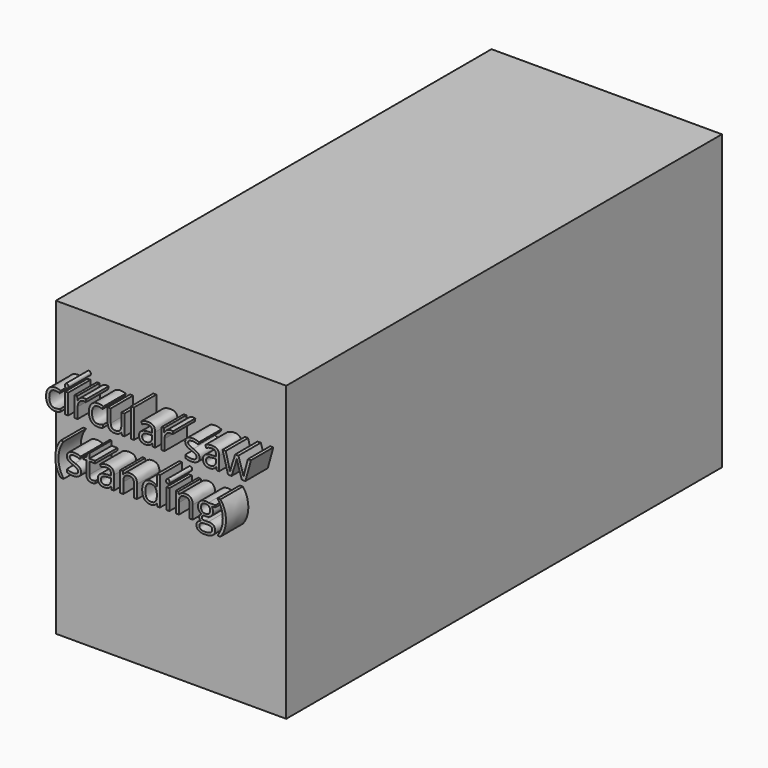
from build123d import *

# Parameters (mm, degrees)
F0_W         = 209.55
F0_H         = 266.7
F1_DEPTH     = 495.3
F2_TEXT_SIZE = 34.2049152733
F3_DEPTH     = 25.4


# Not quite as in the source:
# - Text() gives the source's letters only with a copy of the font that has no kerning and outlines rounded to 1/6400 em; it was checked with that copy


with BuildPart() as f1:
    # F0 (on Front) → F1 (new body)
    with BuildSketch(Plane.XZ):
        Rectangle(F0_W, F0_H)
    extrude(amount=F1_DEPTH)

    # F2 (on face) → F3 (join)
    with BuildSketch(Plane.XZ.offset(495.3)):
        with Locations((-95.25, 61.8877489649)):
            Text('circular saw', F2_TEXT_SIZE, font='Open Sans', text_align=(TextAlign.LEFT, TextAlign.BOTTOM))
        with Locations((-86.362066547, 15.3690641933)):
            Text('(standing)', F2_TEXT_SIZE, font='Open Sans', text_align=(TextAlign.LEFT, TextAlign.BOTTOM))
    extrude(amount=F3_DEPTH)


solid = f1.part
